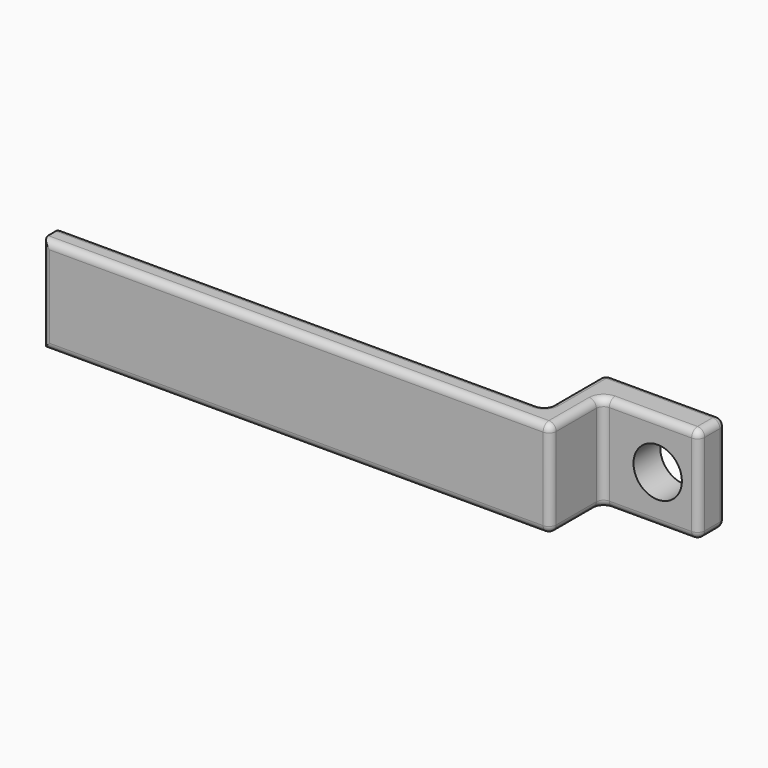
from build123d import *

# Parameters (mm, degrees)
F0_W     = 20
F0_H     = 4
F1_DEPTH = 1
F2_W     = 3.0585520435
F2_H     = 4
F2_W_2   = 1
F3_DEPTH = 1
F4_W     = 1.3837967999
F4_H     = 4
F5_DEPTH = 4
F6_R     = 1
F7_DEPTH = 2
F8_F1_R  = 0.3
F8_F2_R  = 0.3


with BuildPart() as f1:
    # F0 (on Front) → F1 (new body)
    with BuildSketch(Plane.XZ):
        with Locations((-10, 2)):
            Rectangle(F0_W, F0_H)
    extrude(amount=F1_DEPTH)

    # F2 (on face) → F3 (join)
    with BuildSketch(Plane.YZ):
        with Locations((1.5292760218, 2)):
            Rectangle(F2_W, F2_H)
        with Locations((-0.5, 2)):
            Rectangle(F2_W_2, F2_H)
    extrude(amount=F3_DEPTH)

    # F4 (on face) → F5 (join)
    with BuildSketch(Plane.YZ.offset(1)):
        with Locations((2.3666536435, 2)):
            Rectangle(F4_W, F4_H)
    extrude(amount=F5_DEPTH)

    # F6 (on face) → F7 (cut)
    with BuildSketch(Plane.XZ.offset(-1.6747552436)):
        with Locations((3.2954369672, 2)):
            Circle(F6_R)
    extrude(amount=-F7_DEPTH, mode=Mode.SUBTRACT)

    # F8: fillet of radius 0.3 on 18 edges, made by hand

    # F8_f1
    f8_f1_edges = [f1.edges().sort_by_distance(p)[0] for p in [
        (0, 0, 2),
        (1, 1.6747552436, 2),
    ]]
    fillet(f8_f1_edges, radius=F8_F1_R)

    # F8_f2
    f8_f2_edges = [f1.edges().sort_by_distance(p)[0] for p in [
        (-9.5, -1, 0),
        (1, -1, 2),
        (-9.5, -1, 4),
        (-20, -1, 2),
        (-10.15, 0, 0),
        (-10.15, 0, 4),
        (-20, 0, 2),
        (2.5, 3.0585520435, 0),
        (2.5, 3.0585520435, 4),
        (5, 3.0585520435, 2),
        (0, 3.0585520435, 2),
        (5, 1.6747552436, 2),
        (5, 2.3666536435, 0),
        (5, 2.3666536435, 4),
        (3.15, 1.6747552436, 0),
        (3.15, 1.6747552436, 4),
        (1.0878679656, 1.5868872779, 4),
        (1.0878679656, 1.5868872779, 0),
        (-0.0878679656, 0.0878679656, 4),
        (-0.0878679656, 0.0878679656, 0),
    ]]
    fillet(f8_f2_edges, radius=F8_F2_R)


solid = f1.part
